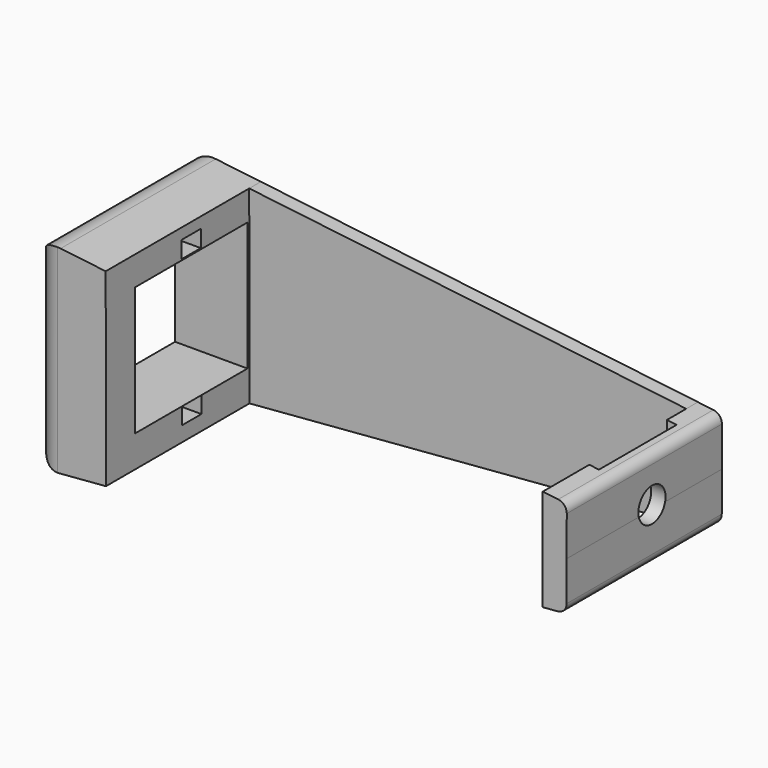
from build123d import *

# Parameters (mm, degrees)
F1_DEPTH  = 40
F3_DEPTH  = 37
F5_DEPTH  = 25
F6_R      = 5
F7_R      = 2
F9_W      = 5
F9_H      = 3.5
F9_H_2    = 3.4365921294
F10_DEPTH = 10
F11_W     = 20
F11_H     = 20.9946793665
F12_DEPTH = 2
F13_R     = 3.5
F14_DEPTH = 25


with BuildPart() as f1:
    # F0 (on Front) → F1 (new body)
    with BuildSketch(Plane.XZ):
        Polygon((-35.1044990334, 40.2309528088), (-35.0494137004, 1.2149916954), (54.9756615806, 8.540398173), (55.0351284044, 29.5349933202), align=None)
        Polygon((-49.999999976, 41.9984515125), (-49.999999976, -0.0015484875), (-35.0494137004, 1.2149916954), (-35.1044990334, 40.2309528088), align=None)
        Polygon((55.0351284044, 29.5349933202), (54.9756615806, 8.540398173), (59.9591903392, 8.9459115673), (59.9591903392, 18.9459115673), (60.0002953853, 28.9458270857), align=None)
    extrude(amount=F1_DEPTH)

    # F2 (on face) → F3 (cut)
    with BuildSketch(Plane.XZ.offset(40)):
        Polygon((-35.1044990334, 40.2309528088), (-35.0494137004, 1.2149916954), (54.9756615806, 8.540398173), (55.0351284044, 29.5349933202), align=None)
    extrude(amount=-F3_DEPTH, mode=Mode.SUBTRACT)

    # F4 (on face) → F5 (cut)
    with BuildSketch(Plane(origin=(-49.999999976, 0, 0), x_dir=(0, -1, 0), z_dir=(-1, 0, 0))):
        Polygon((3.5, 34.2484515125), (3.5, 20.9984515125), (3.5, 7.7484515125), (32.5, 7.7484515125), (32.5, 34.2484515125), align=None)
    extrude(amount=-F5_DEPTH, mode=Mode.SUBTRACT)

    # F6
    f6_edges = [f1.edges().sort_by_distance(p)[0] for p in [
        (-50, -20, 41.998452),
        (-50, -20, -0.001548),
        (-50, -40, 20.998452),
    ]]
    fillet(f6_edges, radius=F6_R)

    # F7
    f7_edges = [f1.edges().sort_by_distance(p)[0] for p in [
        (60.000295, -20, 28.945827),
        (59.95919, -20, 8.945912),
    ]]
    fillet(f7_edges, radius=F7_R)

    # F9 (on face) → F10 (cut)
    with BuildSketch(Plane(origin=(-35.0476284314, 0, -0.0494825765), x_dir=(0, 1, 0), z_dir=(0.9999990033, 0, 0.0014118652))):
        with Locations((-17.9936658144, 36.2820627093)):
            Rectangle(F9_W, F9_H)
        with Locations((-17.8817171156, 6.0796457964)):
            Rectangle(F9_W, F9_H_2)
    extrude(amount=-F10_DEPTH, mode=Mode.SUBTRACT)

    # F11 (on face) → F12 (cut)
    with BuildSketch(Plane(origin=(54.9510301824, 0, -0.1556478324), x_dir=(0, -1, 0), z_dir=(-0.9999959885, 0, 0.0028324712))):
        with Locations((18, 19.1934205725)):
            Rectangle(F11_W, F11_H)
    extrude(amount=-F12_DEPTH, mode=Mode.SUBTRACT)

    # F13 (on face) → F14 (cut)
    with BuildSketch(Plane(origin=(56.9510221594, 0, -0.1613127747), x_dir=(0, -1, 0), z_dir=(-0.9999959885, 0, 0.0028324712))):
        with Locations((18, 19.9799891561)):
            Circle(F13_R)
    extrude(amount=-F14_DEPTH, mode=Mode.SUBTRACT)


solid = f1.part
